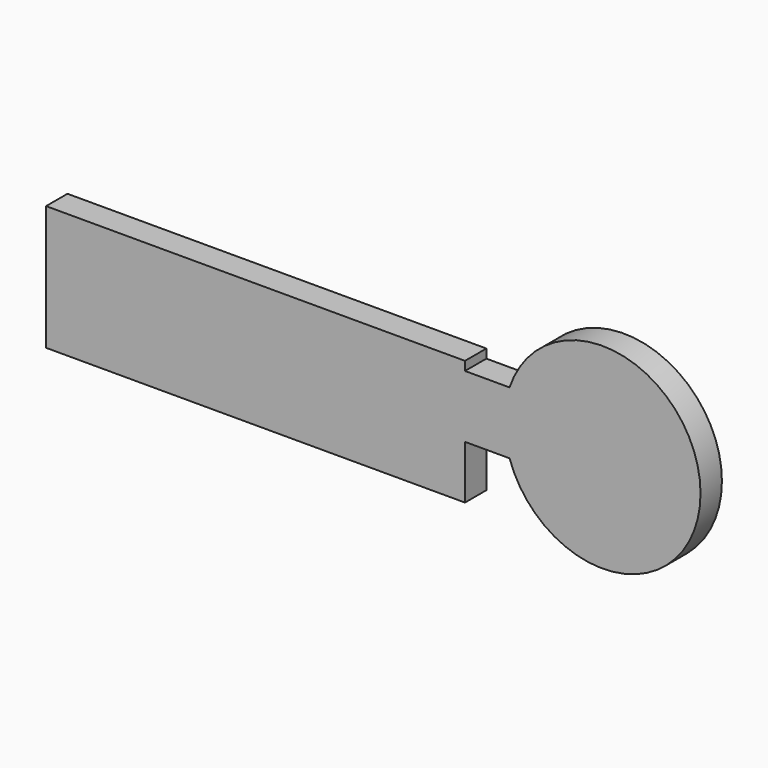
from build123d import *

# Parameters (mm, degrees)
F0_W     = 5
F0_H     = 7
F0_R     = 3
F1_DEPTH = 3


# Not quite as in the source:
# - a feature names something its author has since deleted; it is built from what else it names


with BuildPart() as f1:
    # F0 (on Front) → F1 (new body)
    with BuildSketch(Plane.XZ):
        Polygon((1.3333333333, 0), (0, 0), (0, 7), (-10, 2.5), (-10, -2), (-2, -2), align=None)
        Polygon((0, 7), (0, 0), (1.3333333333, 0), (8, 4), (13, 4), (14.2307692308, 0), (32, 0), (35, 0), (35, 7), align=None)
        Polygon((32, 0), (14.2307692308, 0), (15, -2.5), (11.75, -3.5), (15, -5), align=None)
        with Locations((37.5, 3.5)):
            Rectangle(F0_W, F0_H)
        with BuildLine():
            ThreePointArc((40, 0), (61.4283268073, 3.5), (40, 7))
            Line((40, 7), (40, 0))
        make_face()
        with Locations((57.4283268073, 3.5)):
            Circle(F0_R, mode=Mode.SUBTRACT)
        Polygon((8, 4), (1.3333333333, 0), (14.2307692308, 0), (13, 4), align=None)
        Polygon((14.2307692308, 0), (1.3333333333, 0), (-2, -2), (-10, -2), (-10, 2.5), (0, 7), (35, 7), (35, 8), (-12, 8), (-12, -6), (35, -6), (35, 0), (32, 0), (15, -5), (11.75, -3.5), (15, -2.5), align=None)
        with Locations((57.4283268073, 3.5)):
            Circle(F0_R)
    extrude(amount=F1_DEPTH)


solid = f1.part
